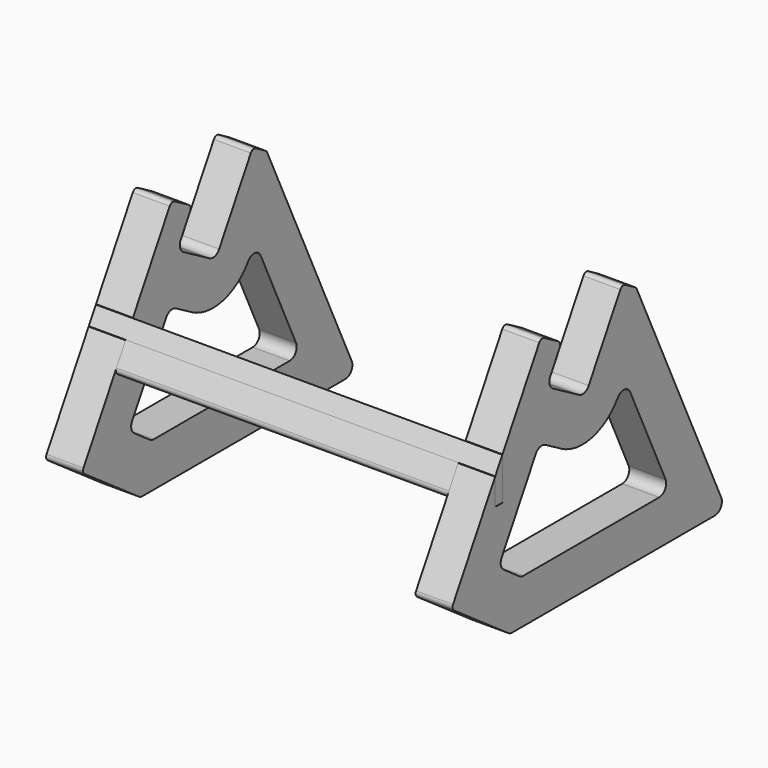
from build123d import *

# Parameters (mm, degrees)
F1_DEPTH = 10
F3_DEPTH = 110
F6_DEPTH = 90


with BuildPart() as f1:
    # F0 (on Right) → F1 (new body)
    with BuildSketch(Plane.YZ):
        with BuildLine():
            ThreePointArc((-36.7022250411, 14.8401355158), (-36.8345497651, 13.9804079791), (-36.3512862802, 13.2571530627))
            Line((-36.3512862802, 13.2571530627), (-18.0379759126, 0.4340350937))
            ThreePointArc((-18.0379759126, 0.4340350937), (-17.3830863842, 0.1110793182), (-16.6613924654, 0))
            Line((-16.6613924654, 0), (-10.9696551146, 0))
            Line((-10.9696551146, 0), (21.5004440397, 0))
            Line((21.5004440397, 0), (51.8494393291, 0))
            ThreePointArc((51.8494393291, 0), (53.873578799, 1.11048094), (54.0245780179, 3.4142838282))
            Line((54.0245780179, 3.4142838282), (28.5975649026, 57.9426894219))
            Line((28.5975649026, 57.9426894219), (25.3900549102, 64.8212167982))
            ThreePointArc((25.3900549102, 64.8212167982), (25.1872183699, 65.1247831332), (24.9024855658, 65.3533053686))
            Line((24.9024855658, 65.3533053686), (21.5296115413, 67.3006350946))
            ThreePointArc((21.5296115413, 67.3006350946), (20.6190286872, 67.4205156016), (19.8903810568, 66.8614046101))
            Line((19.8903810568, 66.8614046101), (15.0818577539, 58.5327979401))
            Line((15.0818577539, 58.5327979401), (9.1903810568, 48.3284609691))
            ThreePointArc((9.1903810568, 48.3284609691), (7.7330857959, 47.210238986), (5.9119200877, 47.45))
            Line((5.9119200877, 47.45), (-2.9215390309, 52.55))
            ThreePointArc((-2.9215390309, 52.55), (-4.039761014, 54.0072952608), (-3.8, 55.8284609691))
            Line((-3.8, 55.8284609691), (-0.6, 61.3710235533))
            ThreePointArc((-0.6, 61.3710235533), (-0.480119493, 62.2816064074), (-1.0392304845, 63.0102540378))
            Line((-1.0392304845, 63.0102540378), (-5.8607235087, 65.7939443332))
            ThreePointArc((-5.8607235087, 65.7939443332), (-6.7960585918, 65.917083533), (-7.5445129349, 65.3427743163))
            Line((-7.5445129349, 65.3427743163), (-19.9782563746, 43.8068989504))
            Line((-19.9782563746, 43.8068989504), (-19.9782563746, 32.2560444474))
            Line((-19.9782563746, 32.2560444474), (-22.4782563746, 32.2560444474))
            Line((-22.4782563746, 32.2560444474), (-22.4782563746, 39.4767719315))
            Line((-22.4782563746, 39.4767719315), (-36.7022250411, 14.8401355158))
        make_face()
        with BuildLine():
            Line((33.0132124036, 12), (-12.8778069988, 12))
            ThreePointArc((-12.8778069988, 12), (-13.5995009176, 12.1110793182), (-14.2543904461, 12.4340350937))
            Line((-14.2543904461, 12.4340350937), (-19.5602569253, 16.1492427992))
            ThreePointArc((-19.5602569253, 16.1492427992), (-20.5267838952, 17.5957526321), (-20.2621344472, 19.3152077055))
            Line((-20.2621344472, 19.3152077055), (-8.7358983849, 39.2792341855))
            ThreePointArc((-8.7358983849, 39.2792341855), (-7.278603124, 40.3974561686), (-5.4574374158, 40.1576951546))
            Line((-5.4574374158, 40.1576951546), (-0.0880799123, 37.0576951546))
            ThreePointArc((-0.0880799123, 37.0576951546), (10.3395153002, 35.4948360224), (19.0366165588, 41.456186564))
            ThreePointArc((19.0366165588, 41.456186564), (21.2143626616, 42.5032512616), (23.1992046596, 41.1250913247))
            Line((23.1992046596, 41.1250913247), (35.1883510925, 15.4142838282))
            ThreePointArc((35.1883510925, 15.4142838282), (35.0373518736, 13.11048094), (33.0132124036, 12))
        make_face(mode=Mode.SUBTRACT)
    extrude(amount=F1_DEPTH)


with BuildPart() as f3:
    # F2 (on face) → F3 (new body)
    with BuildSketch(Plane(origin=(0, 0, 0), x_dir=(0, -1, 0), z_dir=(-1, 0, 0))):
        Polygon((20.0282563746, 32.3060444474), (22.4282563746, 32.3060444474), (22.4282563746, 39.5633744719), (20.0282563746, 43.72029641), align=None)
    extrude(amount=-F3_DEPTH)

    # F5 (on offset) → F6 (join)
    with BuildSketch(Plane(origin=(10, 0, 0), x_dir=(0, -1, 0), z_dir=(-1, 0, 0))):
        with BuildLine():
            Line((22.4282563746, 39.5633744719), (22.4282563746, 32.3060444474))
            Line((22.4282563746, 32.3060444474), (24.5398168487, 32.3060444474))
            ThreePointArc((24.5398168487, 32.3060444474), (25.5790473333, 32.9060444474), (25.5790473333, 34.1060444474))
            Line((25.5790473333, 34.1060444474), (22.4282563746, 39.5633744719))
        make_face()
    extrude(amount=-F6_DEPTH)


with BuildPart() as f7_1:
    # F7: copy of F1
    add(f1.part.moved(Location((100, 0, 0))))


solid = Compound([f1.part, f3.part, f7_1.part])
